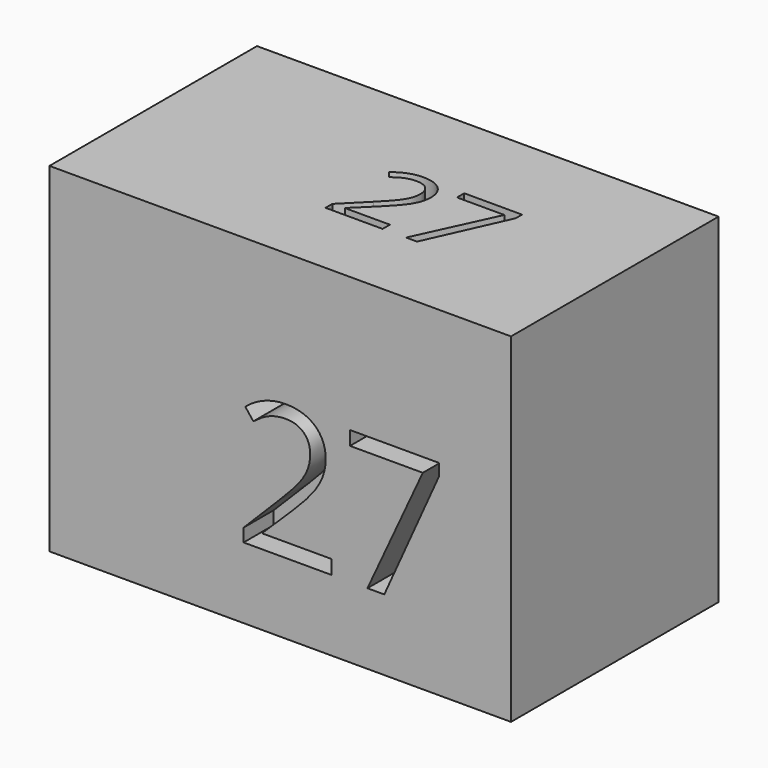
from build123d import *

# Parameters (mm, degrees)
F0_W         = 306
F0_H         = 172
F1_DEPTH     = 225
F2_TEXT_SIZE = 124.0650140163
F3_DEPTH     = 25
F4_TEXT_SIZE = 80.6855141289
F5_DEPTH     = 25


# Not quite as in the source:
# - Text() gives the source's letters only with a copy of the font that has no kerning and outlines rounded to 1/6400 em; it was checked with that copy


with BuildPart() as f1:
    # F0 (on Top) → F1 (new body)
    with BuildSketch(Plane.XY):
        with Locations((153, 86)):
            Rectangle(F0_W, F0_H)
    extrude(amount=F1_DEPTH)

    # F2 (on face) → F3 (cut)
    with BuildSketch(Plane.XZ):
        with Locations((122.6324439049, 47.0795072615)):
            Text('27', F2_TEXT_SIZE, font='Open Sans', text_align=(TextAlign.LEFT, TextAlign.BOTTOM))
    extrude(amount=-F3_DEPTH, mode=Mode.SUBTRACT)

    # F4 (on face) → F5 (cut)
    with BuildSketch(Plane.XY.offset(225)):
        with Locations((137.0141580701, 52.573621273)):
            Text('27', F4_TEXT_SIZE, font='Open Sans', text_align=(TextAlign.LEFT, TextAlign.BOTTOM))
    extrude(amount=-F5_DEPTH, mode=Mode.SUBTRACT)


solid = f1.part
